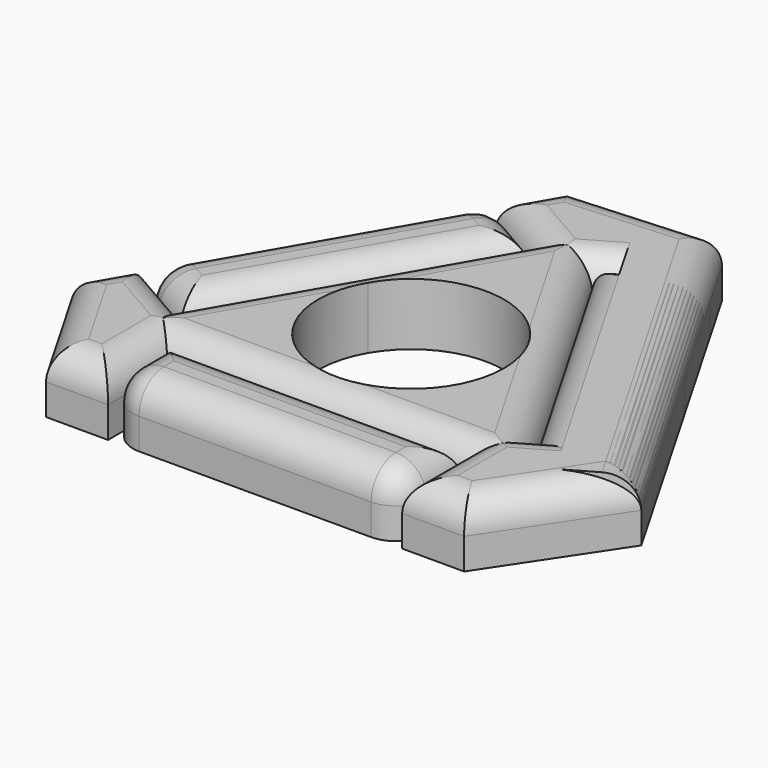
from build123d import *

# Parameters (mm, degrees)
F1_DEPTH       = 10
F2_DEPTH       = 10
F3_DEPTH       = 10
F0_W           = 47.4536935985
F0_H           = 4
F0_H_2         = 8
F4_DEPTH       = 10
F5_T1_DEPTH    = 82.4536935985
F5_T3_DEPTH    = 17.5
F5_T5_DEPTH    = 64.9536935985
F5_T7_DEPTH    = 22.5
F5_S11_W       = 5
F5_S11_H       = 5
F5_T12_DEPTH   = 5
F5_2_T1_DEPTH  = 72.4536935985
F5_2_T3_DEPTH  = 17.5
F5_2_T5_DEPTH  = 19.5
F5_2_T7_DEPTH  = 37.4536935985
F5_2_T9_DEPTH  = 19.5
F5_2_S13_W     = 5
F5_2_S13_H     = 5
F5_2_T14_DEPTH = 5
F5_2_S19_W     = 5
F5_2_S19_H     = 5
F5_2_T20_DEPTH = 5
F5_3_T1_DEPTH  = 47.4536935985
F5_3_T3_DEPTH  = 24.5
F5_3_T5_DEPTH  = 24.5
F5_3_T7_DEPTH  = 47.4536935985
F5_3_T9_DEPTH  = 24.5
F5_3_T11_DEPTH = 35
F5_3_T13_DEPTH = 45.7846096908
F5_3_T15_DEPTH = 35
F5_3_T17_DEPTH = 35
F5_3_T19_DEPTH = 48.4307490277
F5_3_T21_DEPTH = 92.4536935985
F5_3_T23_DEPTH = 48.4307490277
F5_3_T25_DEPTH = 35
F5_3_T27_DEPTH = 47.4536935985
F5_3_T29_DEPTH = 4
F5_3_T31_DEPTH = 4
F5_3_T37_DEPTH = 37
F5_3_T41_DEPTH = 59.9536935985
F5_3_T48_DEPTH = 37
F5_3_T52_DEPTH = 59.9536935985
F5_3_T59_DEPTH = 37
F5_3_T63_DEPTH = 59.9536935985
F5_3_T70_DEPTH = 59.9536935985
F5_3_T74_DEPTH = 37
F5_3_T81_DEPTH = 59.9536935985
F5_3_T85_DEPTH = 16.5
F5_3_T92_DEPTH = 59.9536935985
F5_3_T96_DEPTH = 16.5
F5_4_T1_DEPTH  = 72.4536935985
F5_4_T3_DEPTH  = 17.5
F5_4_T5_DEPTH  = 37.4536935985
F5_4_T7_DEPTH  = 19.5
F5_4_S11_W     = 5
F5_4_S11_H     = 5
F5_4_T12_DEPTH = 5
F5_4_S17_W     = 5
F5_4_S17_H     = 5
F5_4_T18_DEPTH = 5


# Not quite as in the source:
# - a fillet or chamfer that OpenCascade refuses, or shapes differently, is made with other operations: its cross-section is extruded or revolved along the edge and cut away or added
# - two fillets or chamfers of one size are made in one step


with BuildPart() as f1:
    # F0 (on Top) → F1 (new body)
    with BuildSketch(Plane.XY):
        Polygon((-23.7268467993, 0), (-33.7268467993, 0), (-33.7268467993, -12), (-23.7268467993, -12), (-23.7268467993, -4), align=None)
        Polygon((33.7268467993, 0), (23.7268467993, 0), (23.7268467993, -4), (23.7268467993, -12), (33.7268467993, -12), align=None)
        Polygon((46.717227856, 7.5), (33.7268467993, 0), (33.7268467993, -12), align=None)
        Polygon((28.7268467993, 8.6602540378), (33.7268467993, 0), (46.717227856, 7.5), (17.9903810568, 57.2563581976), (8.4641016151, 51.7563581976), (32.1909484144, 10.6602540378), align=None)
        Polygon((12.9903810568, 65.9166122354), (0, 58.4166122354), (5, 49.7563581976), (8.4641016151, 51.7563581976), (17.9903810568, 57.2563581976), align=None)
        Polygon((-10.3923048454, 64.4166122354), (0, 58.4166122354), (12.9903810568, 65.9166122354), align=None)
        Polygon((-8.4641016151, 51.7563581976), (-5, 49.7563581976), (0, 58.4166122354), (-10.3923048454, 64.4166122354), (-15.3923048454, 55.7563581976), align=None)
        Polygon((-44.1191516447, 6), (-33.7268467993, 0), (-28.7268467993, 8.6602540378), (-32.1909484144, 10.6602540378), (-39.1191516447, 14.6602540378), align=None)
        Polygon((-33.7268467993, -12), (-33.7268467993, 0), (-44.1191516447, 6), align=None)
        with BuildLine():
            Line((-5, 49.7563581976), (-16.8634233996, 29.2083061177))
            Line((-16.8634233996, 29.2083061177), (-12.9903810568, 26.9722040785))
            ThreePointArc((-12.9903810568, 26.9722040785), (0, 34.4722040785), (12.9903810568, 26.9722040785))
            Line((12.9903810568, 26.9722040785), (16.8634233996, 29.2083061177))
            Line((16.8634233996, 29.2083061177), (5, 49.7563581976))
            Line((5, 49.7563581976), (0, 58.4166122354))
            Line((0, 58.4166122354), (-5, 49.7563581976))
        make_face()
        with BuildLine():
            Line((-28.7268467993, 8.6602540378), (-33.7268467993, 0))
            Line((-33.7268467993, 0), (-23.7268467993, 0))
            Line((-23.7268467993, 0), (23.7268467993, 0))
            Line((23.7268467993, 0), (33.7268467993, 0))
            Line((33.7268467993, 0), (28.7268467993, 8.6602540378))
            Line((28.7268467993, 8.6602540378), (16.8634233996, 29.2083061177))
            Line((16.8634233996, 29.2083061177), (12.9903810568, 26.9722040785))
            ThreePointArc((12.9903810568, 26.9722040785), (14.4888873943, 23.354489755), (15, 19.4722040785))
            ThreePointArc((15, 19.4722040785), (-3.8822856765, 4.9833166841), (-12.9903810568, 26.9722040785))
            Line((-12.9903810568, 26.9722040785), (-16.8634233996, 29.2083061177))
            Line((-16.8634233996, 29.2083061177), (-28.7268467993, 8.6602540378))
        make_face()
    extrude(amount=F1_DEPTH)

    # F5#3: fillet of radius 5 on 17 edges, made by hand

    # F5_3_s2 → F5_3_t1 (cut)
    with BuildSketch(Plane(origin=(20.2951350994, 35.1522051387, 0), x_dir=(0, 0, 1), z_dir=(-0.5, -0.8660254038, 0))):
        with BuildLine():
            ThreePointArc((5, 29.2083061177), (8.5355339059, 27.7438400236), (10, 24.2083061177))
            Line((10, 24.2083061177), (10, 29.2083061177))
            Line((10, 29.2083061177), (5, 29.2083061177))
        make_face()
    extrude(amount=F5_3_T1_DEPTH, mode=Mode.SUBTRACT)

    # F5_3_s4 → F5_3_t3 (cut)
    with BuildSketch(Plane(origin=(-46.5127574922, 26.8541530589, 0), x_dir=(0, 0, 1), z_dir=(0.8660254038, -0.5, 0))):
        with BuildLine():
            ThreePointArc((5, -40.5902701989), (8.5355339059, -42.0547362929), (10, -45.5902701989))
            Line((10, -45.5902701989), (10, -40.5902701989))
            Line((10, -40.5902701989), (5, -40.5902701989))
        make_face()
    extrude(amount=F5_3_T3_DEPTH, mode=Mode.SUBTRACT)

    # F5_3_s6 → F5_3_t5 (cut)
    with BuildSketch(Plane(origin=(-25.2951350994, 14.6041530589, 0), x_dir=(0, 0, 1), z_dir=(-0.8660254038, 0.5, 0))):
        with BuildLine():
            ThreePointArc((5, -6.8634233996), (8.5355339059, -8.3278894937), (10, -11.8634233996))
            Line((10, -11.8634233996), (10, -6.8634233996))
            Line((10, -6.8634233996), (5, -6.8634233996))
        make_face()
    extrude(amount=F5_3_T5_DEPTH, mode=Mode.SUBTRACT)

    # F5_3_s8 → F5_3_t7 (cut)
    with BuildSketch(Plane.YZ.offset(-23.7268467993)):
        with BuildLine():
            ThreePointArc((0, 5), (1.4644660941, 8.5355339059), (5, 10))
            Line((5, 10), (0, 10))
            Line((0, 10), (0, 5))
        make_face()
    extrude(amount=F5_3_T7_DEPTH, mode=Mode.SUBTRACT)

    # F5_3_s10 → F5_3_t9 (cut)
    with BuildSketch(Plane.XZ):
        with BuildLine():
            ThreePointArc((23.7268467993, 5), (25.1913128933, 8.5355339059), (28.7268467993, 10))
            Line((28.7268467993, 10), (23.7268467993, 10))
            Line((23.7268467993, 10), (23.7268467993, 5))
        make_face()
        with BuildLine():
            ThreePointArc((-23.7268467993, 5), (-25.1913128933, 8.5355339059), (-28.7268467993, 10))
            Line((-28.7268467993, 10), (-23.7268467993, 10))
            Line((-23.7268467993, 10), (-23.7268467993, 5))
        make_face()
    extrude(amount=F5_3_T9_DEPTH, mode=Mode.SUBTRACT)

    # F5_3_s12 → F5_3_t11 (cut)
    with BuildSketch(Plane(origin=(2.8182883002, 4.8814185263, 0), x_dir=(0, 0, 1), z_dir=(-0.5, -0.8660254038, 0))):
        with BuildLine():
            ThreePointArc((5, 41.2083061177), (8.5355339059, 39.7438400236), (10, 36.2083061177))
            Line((10, 36.2083061177), (10, 41.2083061177))
            Line((10, 41.2083061177), (5, 41.2083061177))
        make_face()
    extrude(amount=F5_3_T11_DEPTH, mode=Mode.SUBTRACT)

    # F5_3_s14 → F5_3_t13 (cut)
    with BuildSketch(Plane(origin=(-19.8778641225, 34.4294706062, 0), x_dir=(0, 0, 1), z_dir=(0.5, -0.8660254038, 0))):
        with BuildLine():
            ThreePointArc((5, 35.2083061177), (8.5355339059, 33.7438400236), (10, 30.2083061177))
            Line((10, 30.2083061177), (10, 35.2083061177))
            Line((10, 35.2083061177), (5, 35.2083061177))
        make_face()
    extrude(amount=F5_3_T13_DEPTH, mode=Mode.SUBTRACT)

    # F5_3_s16 → F5_3_t15 (cut)
    with BuildSketch(Plane.YZ.offset(-46.2268467993)):
        with BuildLine():
            ThreePointArc((-12, 5), (-10.5355339059, 8.5355339059), (-7, 10))
            Line((-7, 10), (-12, 10))
            Line((-12, 10), (-12, 5))
        make_face()
    extrude(amount=F5_3_T15_DEPTH, mode=Mode.SUBTRACT)

    # F5_3_s18 → F5_3_t17 (cut)
    with BuildSketch(Plane.YZ.offset(11.2268467993)):
        with BuildLine():
            ThreePointArc((-12, 5), (-10.5355339059, 8.5355339059), (-7, 10))
            Line((-7, 10), (-12, 10))
            Line((-12, 10), (-12, 5))
        make_face()
    extrude(amount=F5_3_T17_DEPTH, mode=Mode.SUBTRACT)

    # F5_3_s20 → F5_3_t19 (cut)
    with BuildSketch(Plane(origin=(-2.100224497, -3.1526694646, 0), x_dir=(0, 0, 1), z_dir=(0.5544159532, 0.8322397196, 0))):
        with BuildLine():
            ThreePointArc((5, 34.7218129606), (8.5355339059, 33.2573468665), (10, 29.7218129606))
            Line((10, 29.7218129606), (10, 34.7218129606))
            Line((10, 34.7218129606), (5, 34.7218129606))
        make_face()
    extrude(amount=F5_3_T19_DEPTH, mode=Mode.SUBTRACT)

    # F5_3_s22 → F5_3_t21 (cut)
    with BuildSketch(Plane(origin=(14.6817116998, -25.4294706062, 0), x_dir=(0, 0, 1), z_dir=(-0.5, 0.8660254038, 0))):
        with BuildLine():
            ThreePointArc((5, 44.2083061177), (8.5355339059, 42.7438400236), (10, 39.2083061177))
            Line((10, 39.2083061177), (10, 44.2083061177))
            Line((10, 44.2083061177), (5, 44.2083061177))
        make_face()
    extrude(amount=F5_3_T21_DEPTH, mode=Mode.SUBTRACT)

    # F5_3_s24 → F5_3_t23 (cut)
    with BuildSketch(Plane(origin=(29.6227232502, 1.9002985825, 0), x_dir=(0, 0, 1), z_dir=(-0.9979487158, -0.06401844, 0))):
        with BuildLine():
            ThreePointArc((5, 64.9497745996), (8.5355339059, 63.4853085056), (10, 59.9497745996))
            Line((10, 59.9497745996), (10, 64.9497745996))
            Line((10, 64.9497745996), (5, 64.9497745996))
        make_face()
    extrude(amount=F5_3_T23_DEPTH, mode=Mode.SUBTRACT)

    # F5_3_s26 → F5_3_t25 (cut)
    with BuildSketch(Plane(origin=(31.5451350994, 54.6377767239, 0), x_dir=(0, 0, 1), z_dir=(-0.5, -0.8660254038, 0))):
        with BuildLine():
            ThreePointArc((5, 41.2083061177), (8.5355339059, 39.7438400236), (10, 36.2083061177))
            Line((10, 36.2083061177), (10, 41.2083061177))
            Line((10, 41.2083061177), (5, 41.2083061177))
        make_face()
    extrude(amount=F5_3_T25_DEPTH, mode=Mode.SUBTRACT)

    # F5_3_s28 → F5_3_t27 (cut)
    with BuildSketch(Plane(origin=(3.4317116998, -5.943899021, 0), x_dir=(0, 0, 1), z_dir=(-0.5, 0.8660254038, 0))):
        with BuildLine():
            ThreePointArc((5, 29.2083061177), (8.5355339059, 27.7438400236), (10, 24.2083061177))
            Line((10, 24.2083061177), (10, 29.2083061177))
            Line((10, 29.2083061177), (5, 29.2083061177))
        make_face()
    extrude(amount=F5_3_T27_DEPTH, mode=Mode.SUBTRACT)

    # F5_3_s30 → F5_3_t29 (cut)
    with BuildSketch(Plane(origin=(25.2951350994, 14.6041530589, 0), x_dir=(0, 0, 1), z_dir=(0.8660254038, 0.5, 0))):
        with BuildLine():
            ThreePointArc((5, -40.5902701989), (8.5355339059, -42.0547362929), (10, -45.5902701989))
            Line((10, -45.5902701989), (10, -40.5902701989))
            Line((10, -40.5902701989), (5, -40.5902701989))
        make_face()
    extrude(amount=F5_3_T29_DEPTH, mode=Mode.SUBTRACT)

    # F5_3_s32 → F5_3_t31 (cut)
    with BuildSketch(Plane(origin=(28.7592367146, 16.6041530589, 0), x_dir=(0, 0, 1), z_dir=(-0.8660254038, -0.5, 0))):
        with BuildLine():
            ThreePointArc((5, -6.8634233996), (8.5355339059, -8.3278894937), (10, -11.8634233996))
            Line((10, -11.8634233996), (10, -6.8634233996))
            Line((10, -6.8634233996), (5, -6.8634233996))
        make_face()
    extrude(amount=F5_3_T31_DEPTH, mode=Mode.SUBTRACT)


with BuildPart() as f2:
    # F0 (on Top) → F2 (new body)
    with BuildSketch(Plane.XY):
        Polygon((16.8634233996, 29.2083061177), (28.7268467993, 8.6602540378), (32.1909484144, 10.6602540378), (8.4641016151, 51.7563581976), (5, 49.7563581976), align=None)
        Polygon((28.7268467993, 8.6602540378), (33.7268467993, 0), (46.717227856, 7.5), (17.9903810568, 57.2563581976), (8.4641016151, 51.7563581976), (32.1909484144, 10.6602540378), align=None)
    extrude(amount=F2_DEPTH)

    # F5: fillet of radius 5 on 4 edges, made by hand

    # F5_s2 → F5_t1 (cut)
    with BuildSketch(Plane(origin=(-26.5451350994, 45.977522686, 0), x_dir=(0, 0, 1), z_dir=(0.5, -0.8660254038, 0))):
        with BuildLine():
            ThreePointArc((5, -29.2083061177), (8.5355339059, -30.6727722118), (10, -34.2083061177))
            Line((10, -34.2083061177), (10, -29.2083061177))
            Line((10, -29.2083061177), (5, -29.2083061177))
        make_face()
    extrude(amount=F5_T1_DEPTH, mode=Mode.SUBTRACT)

    # F5_s4 → F5_t3 (cut)
    with BuildSketch(Plane.XY.offset(-12.5)):
        with BuildLine():
            ThreePointArc((20.4903810568, 52.9262311786), (17.4543492634, 55.2558603101), (13.6602540378, 54.7563581976))
            Line((13.6602540378, 54.7563581976), (17.9903810568, 57.2563581976))
            Line((17.9903810568, 57.2563581976), (20.4903810568, 52.9262311786))
        make_face()
    extrude(amount=F5_T3_DEPTH, mode=Mode.SUBTRACT)

    # F5_s6 → F5_t5 (cut)
    with BuildSketch(Plane(origin=(14.6817116998, -25.4294706062, 0), x_dir=(0, 0, 1), z_dir=(-0.5, 0.8660254038, 0))):
        with BuildLine():
            ThreePointArc((5, 44.2083061177), (8.5355339059, 42.7438400236), (10, 39.2083061177))
            Line((10, 39.2083061177), (10, 44.2083061177))
            Line((10, 44.2083061177), (5, 44.2083061177))
        make_face()
    extrude(amount=F5_T5_DEPTH, mode=Mode.SUBTRACT)

    # F5_s8 → F5_t7 (cut)
    with BuildSketch(Plane(origin=(33.9553891373, 19.6041530589, 0), x_dir=(0, 0, 1), z_dir=(-0.8660254038, -0.5, 0))):
        with BuildLine():
            ThreePointArc((5, 40.5902701989), (8.5355339059, 39.1258041048), (10, 35.5902701989))
            Line((10, 35.5902701989), (10, 40.5902701989))
            Line((10, 40.5902701989), (5, 40.5902701989))
        make_face()
    extrude(amount=F5_T7_DEPTH, mode=Mode.SUBTRACT)


with BuildPart() as f3:
    # F0 (on Top) → F3 (new body)
    with BuildSketch(Plane.XY):
        Polygon((-32.1909484144, 10.6602540378), (-28.7268467993, 8.6602540378), (-16.8634233996, 29.2083061177), (-5, 49.7563581976), (-8.4641016151, 51.7563581976), align=None)
        Polygon((-39.1191516447, 14.6602540378), (-32.1909484144, 10.6602540378), (-8.4641016151, 51.7563581976), (-15.3923048454, 55.7563581976), align=None)
    extrude(amount=F3_DEPTH)

    # F5#2: fillet of radius 5 on 6 edges, made by hand

    # F5_2_s2 → F5_2_t1 (cut)
    with BuildSketch(Plane(origin=(-9.6817116998, -16.7692165683, 0), x_dir=(0, 0, 1), z_dir=(0.5, 0.8660254038, 0))):
        with BuildLine():
            ThreePointArc((5, -29.2083061177), (8.5355339059, -30.6727722118), (10, -34.2083061177))
            Line((10, -34.2083061177), (10, -29.2083061177))
            Line((10, -29.2083061177), (5, -29.2083061177))
        make_face()
    extrude(amount=F5_2_T1_DEPTH, mode=Mode.SUBTRACT)

    # F5_2_s4 → F5_2_t3 (cut)
    with BuildSketch(Plane.XY.offset(-12.5)):
        with BuildLine():
            ThreePointArc((-11.0621778265, 53.2563581976), (-14.856273052, 53.7558603101), (-17.8923048454, 51.4262311786))
            Line((-17.8923048454, 51.4262311786), (-15.3923048454, 55.7563581976))
            Line((-15.3923048454, 55.7563581976), (-11.0621778265, 53.2563581976))
        make_face()
        with BuildLine():
            ThreePointArc((-36.6191516447, 18.9903810568), (-37.1186537572, 15.1962858313), (-34.7890246257, 12.1602540378))
            Line((-34.7890246257, 12.1602540378), (-39.1191516447, 14.6602540378))
            Line((-39.1191516447, 14.6602540378), (-36.6191516447, 18.9903810568))
        make_face()
    extrude(amount=F5_2_T3_DEPTH, mode=Mode.SUBTRACT)

    # F5_2_s6 → F5_2_t5 (cut)
    with BuildSketch(Plane(origin=(-14.4698175521, 8.3541530589, 0), x_dir=(0, 0, 1), z_dir=(-0.8660254038, 0.5, 0))):
        with BuildLine():
            ThreePointArc((5, 40.5902701989), (8.5355339059, 39.1258041048), (10, 35.5902701989))
            Line((10, 35.5902701989), (10, 40.5902701989))
            Line((10, 40.5902701989), (5, 40.5902701989))
        make_face()
    extrude(amount=F5_2_T5_DEPTH, mode=Mode.SUBTRACT)

    # F5_2_s8 → F5_2_t7 (cut)
    with BuildSketch(Plane(origin=(17.7951350994, 30.8220781198, 0), x_dir=(0, 0, 1), z_dir=(-0.5, -0.8660254038, 0))):
        with BuildLine():
            ThreePointArc((5, 41.2083061177), (8.5355339059, 39.7438400236), (10, 36.2083061177))
            Line((10, 36.2083061177), (10, 41.2083061177))
            Line((10, 41.2083061177), (5, 41.2083061177))
        make_face()
    extrude(amount=F5_2_T7_DEPTH, mode=Mode.SUBTRACT)

    # F5_2_s10 → F5_2_t9 (cut)
    with BuildSketch(Plane(origin=(-31.3573129259, 18.1041530589, 0), x_dir=(0, 0, 1), z_dir=(0.8660254038, -0.5, 0))):
        with BuildLine():
            ThreePointArc((5, 6.8634233996), (8.5355339059, 5.3989573056), (10, 1.8634233996))
            Line((10, 1.8634233996), (10, 6.8634233996))
            Line((10, 6.8634233996), (5, 6.8634233996))
        make_face()
    extrude(amount=F5_2_T9_DEPTH, mode=Mode.SUBTRACT)


with BuildPart() as f4:
    # F0 (on Top) → F4 (new body)
    with BuildSketch(Plane.XY):
        with Locations((0, -2)):
            Rectangle(F0_W, F0_H)
        with Locations((0, -8)):
            Rectangle(F0_W, F0_H_2)
    extrude(amount=F4_DEPTH)

    # F5#4: fillet of radius 5 on 6 edges, made by hand

    # F5_4_s2 → F5_4_t1 (cut)
    with BuildSketch(Plane.YZ.offset(-36.2268467993)):
        with BuildLine():
            ThreePointArc((0, 5), (-1.4644660941, 8.5355339059), (-5, 10))
            Line((-5, 10), (0, 10))
            Line((0, 10), (0, 5))
        make_face()
    extrude(amount=F5_4_T1_DEPTH, mode=Mode.SUBTRACT)

    # F5_4_s4 → F5_4_t3 (cut)
    with BuildSketch(Plane.XY.offset(-12.5)):
        with BuildLine():
            ThreePointArc((18.7268467993, -12), (22.2623807052, -10.5355339059), (23.7268467993, -7))
            Line((23.7268467993, -7), (23.7268467993, -12))
            Line((23.7268467993, -12), (18.7268467993, -12))
        make_face()
        with BuildLine():
            ThreePointArc((-23.7268467993, -7), (-22.2623807052, -10.5355339059), (-18.7268467993, -12))
            Line((-18.7268467993, -12), (-23.7268467993, -12))
            Line((-23.7268467993, -12), (-23.7268467993, -7))
        make_face()
    extrude(amount=F5_4_T3_DEPTH, mode=Mode.SUBTRACT)

    # F5_4_s6 → F5_4_t5 (cut)
    with BuildSketch(Plane.YZ.offset(-18.7268467993)):
        with BuildLine():
            ThreePointArc((-12, 5), (-10.5355339059, 8.5355339059), (-7, 10))
            Line((-7, 10), (-12, 10))
            Line((-12, 10), (-12, 5))
        make_face()
    extrude(amount=F5_4_T5_DEPTH, mode=Mode.SUBTRACT)

    # F5_4_s8 → F5_4_t7 (cut)
    with BuildSketch(Plane.XZ.offset(-12.5)):
        with BuildLine():
            ThreePointArc((23.7268467993, 5), (22.2623807052, 8.5355339059), (18.7268467993, 10))
            Line((18.7268467993, 10), (23.7268467993, 10))
            Line((23.7268467993, 10), (23.7268467993, 5))
        make_face()
        with BuildLine():
            ThreePointArc((-23.7268467993, 5), (-22.2623807052, 8.5355339059), (-18.7268467993, 10))
            Line((-18.7268467993, 10), (-23.7268467993, 10))
            Line((-23.7268467993, 10), (-23.7268467993, 5))
        make_face()
    extrude(amount=F5_4_T7_DEPTH, mode=Mode.SUBTRACT)


with BuildPart() as f5_tool10:
    # F5_s11 → F5_t12 (new body)
    with BuildSketch(Plane(origin=(33.9553891373, 19.6041530589, 0), x_dir=(0, 0, 1), z_dir=(0.8660254038, 0.5, 0))):
        with Locations((7.5, -38.0902701989)):
            Rectangle(F5_S11_W, F5_S11_H)
    extrude(amount=F5_T12_DEPTH)

    # F5_s13 → F5_t14 (revolve, cut)
    with BuildSketch(Plane(origin=(16.1602540378, 50.4262311786, 5), x_dir=(0.3535533906, -0.6123724357, -0.7071067812), z_dir=(0.3535533906, -0.6123724357, 0.7071067812))):
        with BuildLine():
            ThreePointArc((0, -5), (5, 0), (0, 5))
            Line((0, 5), (0, -5))
        make_face()
    revolve(axis=Axis((16.1602540378, 50.4262311786, 5), (0.8660254038, 0.5, 0)), mode=Mode.SUBTRACT)


with BuildPart() as f2_1:
    add(f2.part)

    # F5_t9: cut F5_tool10
    add(f5_tool10.part, mode=Mode.SUBTRACT)


with BuildPart() as f5_2_tool12:
    # F5_2_s13 → F5_2_t14 (new body)
    with BuildSketch(Plane(origin=(17.7951350994, 30.8220781198, 0), x_dir=(0, 0, 1), z_dir=(0.5, 0.8660254038, 0))):
        with Locations((7.5, -38.7083061177)):
            Rectangle(F5_2_S13_W, F5_2_S13_H)
    extrude(amount=F5_2_T14_DEPTH)

    # F5_2_s15 → F5_2_t16 (revolve, cut)
    with BuildSketch(Plane(origin=(-13.5621778265, 48.9262311786, 5), x_dir=(0.6123724357, -0.3535533906, -0.7071067812), z_dir=(0.6123724357, -0.3535533906, 0.7071067812))):
        with BuildLine():
            ThreePointArc((0, -5), (5, 0), (0, 5))
            Line((0, 5), (0, -5))
        make_face()
    revolve(axis=Axis((-13.5621778265, 48.9262311786, 5), (0.5, 0.8660254038, 0)), mode=Mode.SUBTRACT)


with BuildPart() as f3_1:
    add(f3.part)

    # F5_2_t11: cut F5_2_tool12
    add(f5_2_tool12.part, mode=Mode.SUBTRACT)


with BuildPart() as f5_2_tool18:
    # F5_2_s19 → F5_2_t20 (new body)
    with BuildSketch(Plane(origin=(-31.3573129259, 18.1041530589, 0), x_dir=(0, 0, 1), z_dir=(-0.8660254038, 0.5, 0))):
        with Locations((7.5, -4.3634233996)):
            Rectangle(F5_2_S19_W, F5_2_S19_H)
    extrude(amount=F5_2_T20_DEPTH)

    # F5_2_s21 → F5_2_t22 (revolve, cut)
    with BuildSketch(Plane(origin=(-32.2890246257, 16.4903810568, 5), x_dir=(0.3535533906, 0.6123724357, -0.7071067812), z_dir=(0.3535533906, 0.6123724357, 0.7071067812))):
        with BuildLine():
            ThreePointArc((0, -5), (5, 0), (0, 5))
            Line((0, 5), (0, -5))
        make_face()
    revolve(axis=Axis((-32.2890246257, 16.4903810568, 5), (-0.8660254038, 0.5, 0)), mode=Mode.SUBTRACT)


with BuildPart() as f3_2:
    add(f3_1.part)

    # F5_2_t17: cut F5_2_tool18
    add(f5_2_tool18.part, mode=Mode.SUBTRACT)


with BuildPart() as f5_3_tool35:
    # F5_3_s36 → F5_3_t37 (new body)
    with BuildSketch(Plane(origin=(-46.5127574922, 26.8541530589, 0), x_dir=(0, 0, 1), z_dir=(0.8660254038, -0.5, 0))):
        with BuildLine():
            ThreePointArc((5, -40.5902701989), (8.5355339059, -42.0547362929), (10, -45.5902701989))
            Line((10, -45.5902701989), (10, -40.5902701989))
            Line((10, -40.5902701989), (5, -40.5902701989))
        make_face()
    extrude(amount=F5_3_T37_DEPTH)

    split(bisect_by=Plane(origin=(-25.2951350994, 14.6041530589, 0), x_dir=(0, 0, 1), z_dir=(0.8660254038, -0.5, 0)), keep=Keep.TOP)


with BuildPart() as f5_3_tool39:
    # F5_3_s40 → F5_3_t41 (new body)
    with BuildSketch(Plane(origin=(26.5451350994, 45.977522686, 0), x_dir=(0, 0, 1), z_dir=(-0.5, -0.8660254038, 0))):
        with BuildLine():
            ThreePointArc((5, 29.2083061177), (8.5355339059, 27.7438400236), (10, 24.2083061177))
            Line((10, 24.2083061177), (10, 29.2083061177))
            Line((10, 29.2083061177), (5, 29.2083061177))
        make_face()
    extrude(amount=F5_3_T41_DEPTH)

    split(bisect_by=Plane(origin=(20.2951350994, 35.1522051387, 0), x_dir=(0, 0, 1), z_dir=(0.5, 0.8660254038, 0)), keep=Keep.TOP)


with BuildPart() as f5_3_tool35_1:
    add(f5_3_tool35.part)

    # F5_3_t43: intersect F5_3_tool39
    add(f5_3_tool39.part, mode=Mode.INTERSECT)


with BuildPart() as f1_1:
    add(f1.part)

    # F5_3_t33: cut F5_3_tool35
    add(f5_3_tool35_1.part, mode=Mode.SUBTRACT)


with BuildPart() as f5_3_tool46:
    # F5_3_s47 → F5_3_t48 (new body)
    with BuildSketch(Plane(origin=(-14.4698175521, 8.3541530589, 0), x_dir=(0, 0, 1), z_dir=(-0.8660254038, 0.5, 0))):
        with BuildLine():
            ThreePointArc((5, -6.8634233996), (8.5355339059, -8.3278894937), (10, -11.8634233996))
            Line((10, -11.8634233996), (10, -6.8634233996))
            Line((10, -6.8634233996), (5, -6.8634233996))
        make_face()
    extrude(amount=F5_3_T48_DEPTH)

    split(bisect_by=Plane(origin=(-25.2951350994, 14.6041530589, 0), x_dir=(0, 0, 1), z_dir=(0.8660254038, -0.5, 0)), keep=Keep.TOP)


with BuildPart() as f5_3_tool50:
    # F5_3_s51 → F5_3_t52 (new body)
    with BuildSketch(Plane(origin=(20.2951350994, 35.1522051387, 0), x_dir=(0, 0, 1), z_dir=(-0.5, -0.8660254038, 0))):
        with BuildLine():
            ThreePointArc((5, 29.2083061177), (8.5355339059, 27.7438400236), (10, 24.2083061177))
            Line((10, 24.2083061177), (10, 29.2083061177))
            Line((10, 29.2083061177), (5, 29.2083061177))
        make_face()
    extrude(amount=F5_3_T52_DEPTH)

    split(bisect_by=Plane(origin=(-3.4317116998, -5.943899021, 0), x_dir=(0, 0, 1), z_dir=(-0.5, -0.8660254038, 0)), keep=Keep.TOP)


with BuildPart() as f5_3_tool46_1:
    add(f5_3_tool46.part)

    # F5_3_t54: intersect F5_3_tool50
    add(f5_3_tool50.part, mode=Mode.INTERSECT)


with BuildPart() as f1_2:
    add(f1_1.part)

    # F5_3_t44: cut F5_3_tool46
    add(f5_3_tool46_1.part, mode=Mode.SUBTRACT)


with BuildPart() as f5_3_tool57:
    # F5_3_s58 → F5_3_t59 (new body)
    with BuildSketch(Plane.XZ.offset(24.5)):
        with BuildLine():
            ThreePointArc((-23.7268467993, 5), (-25.1913128933, 8.5355339059), (-28.7268467993, 10))
            Line((-28.7268467993, 10), (-23.7268467993, 10))
            Line((-23.7268467993, 10), (-23.7268467993, 5))
        make_face()
    extrude(amount=-F5_3_T59_DEPTH)

    split(bisect_by=Plane.XZ, keep=Keep.BOTTOM)


with BuildPart() as f5_3_tool61:
    # F5_3_s62 → F5_3_t63 (new body)
    with BuildSketch(Plane.YZ.offset(-36.2268467993)):
        with BuildLine():
            ThreePointArc((0, 5), (1.4644660941, 8.5355339059), (5, 10))
            Line((5, 10), (0, 10))
            Line((0, 10), (0, 5))
        make_face()
    extrude(amount=F5_3_T63_DEPTH)

    split(bisect_by=Plane.YZ.offset(-23.7268467993), keep=Keep.BOTTOM)


with BuildPart() as f5_3_tool57_1:
    add(f5_3_tool57.part)

    # F5_3_t65: intersect F5_3_tool61
    add(f5_3_tool61.part, mode=Mode.INTERSECT)


with BuildPart() as f1_3:
    add(f1_2.part)

    # F5_3_t55: cut F5_3_tool57
    add(f5_3_tool57_1.part, mode=Mode.SUBTRACT)


with BuildPart() as f5_3_tool68:
    # F5_3_s69 → F5_3_t70 (new body)
    with BuildSketch(Plane.YZ.offset(-23.7268467993)):
        with BuildLine():
            ThreePointArc((0, 5), (1.4644660941, 8.5355339059), (5, 10))
            Line((5, 10), (0, 10))
            Line((0, 10), (0, 5))
        make_face()
    extrude(amount=F5_3_T70_DEPTH)

    split(bisect_by=Plane.YZ.offset(23.7268467993), keep=Keep.TOP)


with BuildPart() as f5_3_tool72:
    # F5_3_s73 → F5_3_t74 (new body)
    with BuildSketch(Plane.XZ.offset(-12.5)):
        with BuildLine():
            ThreePointArc((23.7268467993, 5), (25.1913128933, 8.5355339059), (28.7268467993, 10))
            Line((28.7268467993, 10), (23.7268467993, 10))
            Line((23.7268467993, 10), (23.7268467993, 5))
        make_face()
    extrude(amount=F5_3_T74_DEPTH)

    split(bisect_by=Plane.XZ, keep=Keep.BOTTOM)


with BuildPart() as f5_3_tool68_1:
    add(f5_3_tool68.part)

    # F5_3_t76: intersect F5_3_tool72
    add(f5_3_tool72.part, mode=Mode.INTERSECT)


with BuildPart() as f1_4:
    add(f1_3.part)

    # F5_3_t66: cut F5_3_tool68
    add(f5_3_tool68_1.part, mode=Mode.SUBTRACT)


with BuildPart() as f5_3_tool79:
    # F5_3_s80 → F5_3_t81 (new body)
    with BuildSketch(Plane(origin=(9.6817116998, -16.7692165683, 0), x_dir=(0, 0, 1), z_dir=(-0.5, 0.8660254038, 0))):
        with BuildLine():
            ThreePointArc((5, 29.2083061177), (8.5355339059, 27.7438400236), (10, 24.2083061177))
            Line((10, 24.2083061177), (10, 29.2083061177))
            Line((10, 29.2083061177), (5, 29.2083061177))
        make_face()
    extrude(amount=F5_3_T81_DEPTH)

    split(bisect_by=Plane(origin=(3.4317116998, -5.943899021, 0), x_dir=(0, 0, 1), z_dir=(0.5, -0.8660254038, 0)), keep=Keep.TOP)


with BuildPart() as f5_3_tool83:
    # F5_3_s84 → F5_3_t85 (new body)
    with BuildSketch(Plane(origin=(28.7592367146, 16.6041530589, 0), x_dir=(0, 0, 1), z_dir=(-0.8660254038, -0.5, 0))):
        with BuildLine():
            ThreePointArc((5, -6.8634233996), (8.5355339059, -8.3278894937), (10, -11.8634233996))
            Line((10, -11.8634233996), (10, -6.8634233996))
            Line((10, -6.8634233996), (5, -6.8634233996))
        make_face()
    extrude(amount=F5_3_T85_DEPTH)

    split(bisect_by=Plane(origin=(25.2951350994, 14.6041530589, 0), x_dir=(0, 0, 1), z_dir=(-0.8660254038, -0.5, 0)), keep=Keep.TOP)


with BuildPart() as f5_3_tool79_1:
    add(f5_3_tool79.part)

    # F5_3_t87: intersect F5_3_tool83
    add(f5_3_tool83.part, mode=Mode.INTERSECT)


with BuildPart() as f1_5:
    add(f1_4.part)

    # F5_3_t77: cut F5_3_tool79
    add(f5_3_tool79_1.part, mode=Mode.SUBTRACT)


with BuildPart() as f5_3_tool90:
    # F5_3_s91 → F5_3_t92 (new body)
    with BuildSketch(Plane(origin=(3.4317116998, -5.943899021, 0), x_dir=(0, 0, 1), z_dir=(-0.5, 0.8660254038, 0))):
        with BuildLine():
            ThreePointArc((5, 29.2083061177), (8.5355339059, 27.7438400236), (10, 24.2083061177))
            Line((10, 24.2083061177), (10, 29.2083061177))
            Line((10, 29.2083061177), (5, 29.2083061177))
        make_face()
    extrude(amount=F5_3_T92_DEPTH)

    split(bisect_by=Plane(origin=(-20.2951350994, 35.1522051387, 0), x_dir=(0, 0, 1), z_dir=(-0.5, 0.8660254038, 0)), keep=Keep.TOP)


with BuildPart() as f5_3_tool94:
    # F5_3_s95 → F5_3_t96 (new body)
    with BuildSketch(Plane(origin=(14.4698175521, 8.3541530589, 0), x_dir=(0, 0, 1), z_dir=(0.8660254038, 0.5, 0))):
        with BuildLine():
            ThreePointArc((5, -40.5902701989), (8.5355339059, -42.0547362929), (10, -45.5902701989))
            Line((10, -45.5902701989), (10, -40.5902701989))
            Line((10, -40.5902701989), (5, -40.5902701989))
        make_face()
    extrude(amount=F5_3_T96_DEPTH)

    split(bisect_by=Plane(origin=(25.2951350994, 14.6041530589, 0), x_dir=(0, 0, 1), z_dir=(-0.8660254038, -0.5, 0)), keep=Keep.TOP)


with BuildPart() as f5_3_tool90_1:
    add(f5_3_tool90.part)

    # F5_3_t98: intersect F5_3_tool94
    add(f5_3_tool94.part, mode=Mode.INTERSECT)


with BuildPart() as f1_6:
    add(f1_5.part)

    # F5_3_t88: cut F5_3_tool90
    add(f5_3_tool90_1.part, mode=Mode.SUBTRACT)


with BuildPart() as f5_4_tool10:
    # F5_4_s11 → F5_4_t12 (new body)
    with BuildSketch(Plane.XZ.offset(7)):
        with Locations((21.2268467993, 7.5)):
            Rectangle(F5_4_S11_W, F5_4_S11_H)
    extrude(amount=F5_4_T12_DEPTH)

    # F5_4_s13 → F5_4_t14 (revolve, cut)
    with BuildSketch(Plane(origin=(18.7268467993, -7, 5), x_dir=(-0.7071067812, 0, -0.7071067812), z_dir=(-0.7071067812, 0, 0.7071067812))):
        with BuildLine():
            ThreePointArc((0, -5), (5, 0), (0, 5))
            Line((0, 5), (0, -5))
        make_face()
    revolve(axis=Axis((18.7268467993, -7, 5), (0, -1, 0)), mode=Mode.SUBTRACT)


with BuildPart() as f4_1:
    add(f4.part)

    # F5_4_t9: cut F5_4_tool10
    add(f5_4_tool10.part, mode=Mode.SUBTRACT)


with BuildPart() as f5_4_tool16:
    # F5_4_s17 → F5_4_t18 (new body)
    with BuildSketch(Plane.YZ.offset(-18.7268467993)):
        with Locations((-9.5, 7.5)):
            Rectangle(F5_4_S17_W, F5_4_S17_H)
    extrude(amount=-F5_4_T18_DEPTH)

    # F5_4_s19 → F5_4_t20 (revolve, cut)
    with BuildSketch(Plane(origin=(-18.7268467993, -7, 5), x_dir=(0, 0.7071067812, -0.7071067812), z_dir=(0, 0.7071067812, 0.7071067812))):
        with BuildLine():
            ThreePointArc((0, -5), (5, 0), (0, 5))
            Line((0, 5), (0, -5))
        make_face()
    revolve(axis=Axis((-18.7268467993, -7, 5), (-1, 0, 0)), mode=Mode.SUBTRACT)


with BuildPart() as f4_2:
    add(f4_1.part)

    # F5_4_t15: cut F5_4_tool16
    add(f5_4_tool16.part, mode=Mode.SUBTRACT)


solid = Compound([f2_1.part, f3_2.part, f1_6.part, f4_2.part])
